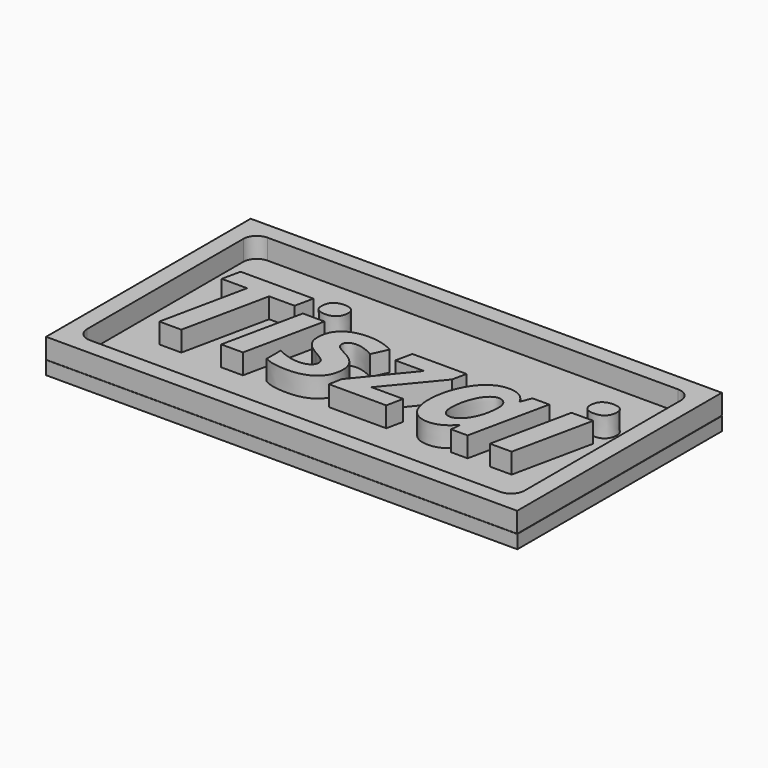
from build123d import *

# Parameters (mm, degrees)
F0_TEXT_SIZE = 21.9466194205
F1_DEPTH     = 3
F0_W         = 70
F0_H         = 38
F2_DEPTH     = 3
F3_W         = 70
F3_H         = 38
F4_DEPTH     = 2


# Not quite as in the source:
# - Text() gives the source's letters only with a copy of the font that has no kerning and outlines rounded to 1/6400 em; it was checked with that copy


with BuildPart() as f1:
    # F0 (on Top) → F1 (new body)
    with BuildSketch(Plane.XY):
        with Locations((-29.2522731619, -9.3339501584)):
            Text('Tiszai', F0_TEXT_SIZE, font='Open Sans', font_style=FontStyle.BOLDITALIC, text_align=(TextAlign.LEFT, TextAlign.BOTTOM))
    extrude(amount=F1_DEPTH)


with BuildPart() as f2:
    # F0 (on Top) → F2 (new body)
    with BuildSketch(Plane.XY):
        with Locations((0.7294841856, -1.5323841757)):
            Rectangle(F0_W, F0_H)
        with BuildLine():
            ThreePointArc((-31.7705158144, 12.9676158243), (-31.1847293768, 14.3818293867), (-29.7705158144, 14.9676158243))
            Line((-29.7705158144, 14.9676158243), (31.2294841856, 14.9676158243))
            ThreePointArc((31.2294841856, 14.9676158243), (32.6436977479, 14.3818293867), (33.2294841856, 12.9676158243))
            Line((33.2294841856, 12.9676158243), (33.2294841856, -16.0323841757))
            ThreePointArc((33.2294841856, -16.0323841757), (32.6436977479, -17.446597738), (31.2294841856, -18.0323841757))
            Line((31.2294841856, -18.0323841757), (-29.7705158144, -18.0323841757))
            ThreePointArc((-29.7705158144, -18.0323841757), (-31.1847293768, -17.446597738), (-31.7705158144, -16.0323841757))
            Line((-31.7705158144, -16.0323841757), (-31.7705158144, 12.9676158243))
        make_face(mode=Mode.SUBTRACT)
    extrude(amount=F2_DEPTH)


with BuildPart() as f4:
    # F3 (on Top) → F4 (new body)
    with BuildSketch(Plane.XY):
        with Locations((0.7863679528, -1.5771289766)):
            Rectangle(F3_W, F3_H)
    extrude(amount=-F4_DEPTH)


solid = Compound([f1.part, f2.part, f4.part])
